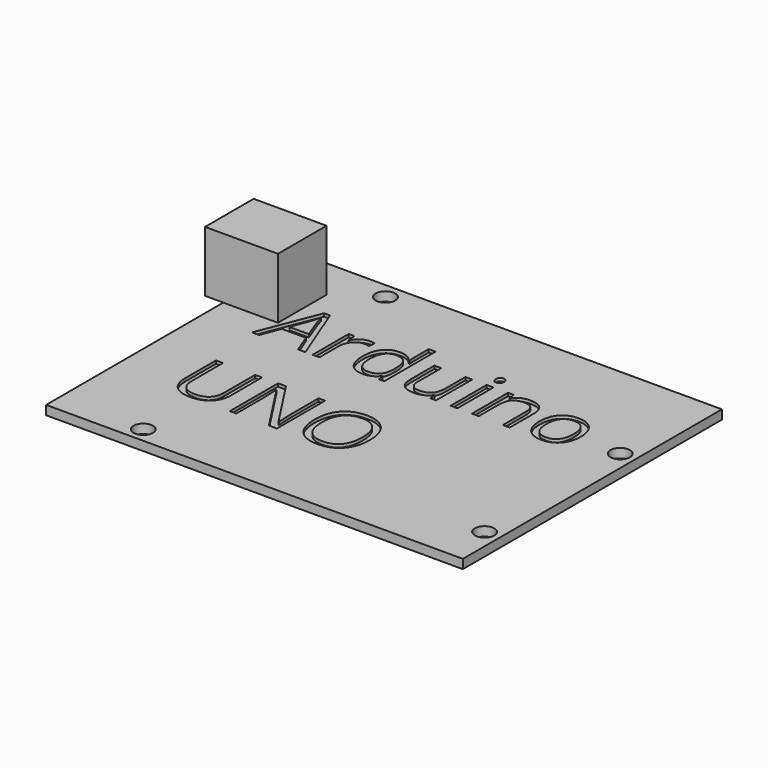
from build123d import *

# Parameters (mm, degrees)
F0_W         = 68.6
F0_H         = 53.3
F0_R         = 1.6
F1_DEPTH     = 1.5
F2_TEXT_SIZE = 13.8888888889
F3_DEPTH     = 0.5
F4_W         = 9
F4_H         = 10
F4_W_2       = 3
F5_DEPTH     = 10


# Not quite as in the source:
# - Text() gives the source's letters only with a copy of the font that has no kerning and outlines rounded to 1/6400 em; it was checked with that copy


with BuildPart() as f1:
    # F0 (on Top) → F1 (new body)
    with BuildSketch(Plane.XY):
        with Locations((34.1914687559, 9.2411806947)):
            Rectangle(F0_W, F0_H)
        with Locations((13.8914687559, -14.9088193053)):
            Circle(F0_R, mode=Mode.SUBTRACT)
        with Locations((65.9914687559, -9.8088193053)):
            Circle(F0_R, mode=Mode.SUBTRACT)
        with Locations((15.1914687559, 33.2911806947)):
            Circle(F0_R, mode=Mode.SUBTRACT)
        with Locations((65.9914687559, 18.0911806947)):
            Circle(F0_R, mode=Mode.SUBTRACT)
    extrude(amount=F1_DEPTH)

    # F2 (on face) → F3 (cut)
    with BuildSketch(Plane.XY.offset(1.5)):
        with Locations((7.9450233746, 14.8798691714)):
            Text('Arduino', F2_TEXT_SIZE, font='Open Sans', text_align=(TextAlign.LEFT, TextAlign.BOTTOM))
        with Locations((7.9450233746, -4.0090197175)):
            Text('UNO', F2_TEXT_SIZE, font='Open Sans', text_align=(TextAlign.LEFT, TextAlign.BOTTOM))
    extrude(amount=-F3_DEPTH, mode=Mode.SUBTRACT)

    # F4 (on face) → F5 (join)
    with BuildSketch(Plane.XY.offset(1.5)):
        with Locations((4.3914687559, 24.0493685752)):
            Rectangle(F4_W, F4_H)
        with Locations((-1.6085312441, 24.0493685752)):
            Rectangle(F4_W_2, F4_H)
    extrude(amount=F5_DEPTH)


solid = f1.part
